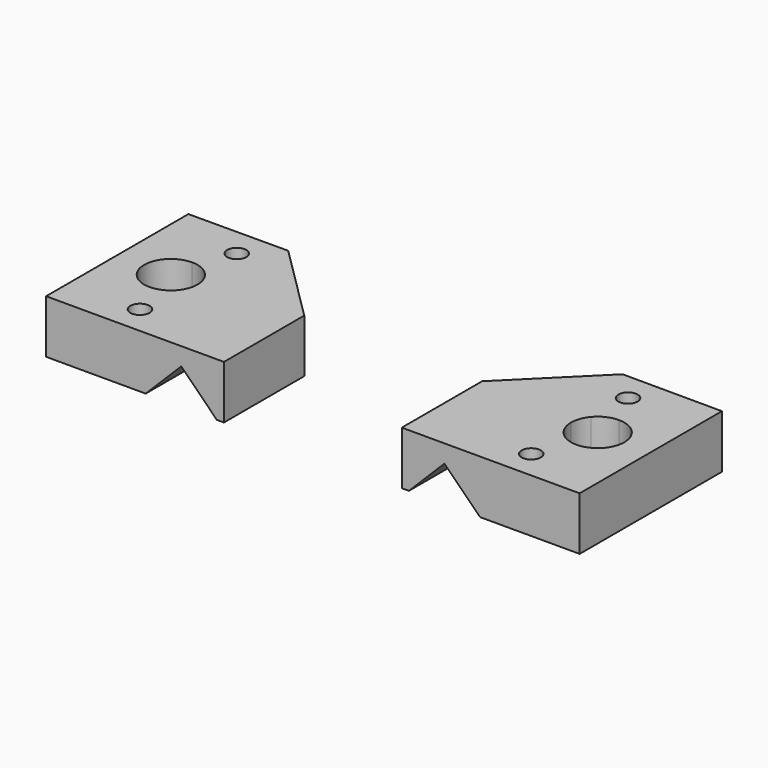
from build123d import *

# Parameters (mm, degrees)
F1_DEPTH  = 15
F3_DEPTH  = 50.1607448159
F4_R      = 4
F5_DEPTH  = 10
F7_DEPTH  = 15.001
F9_D      = 5.4
F9_DEPTH  = 60
F9_TIP    = 1.6223236714
F11_DEPTH = 15.001


with BuildPart() as f1:
    # F0 (on Top) → F1 (new body)
    with BuildSketch(Plane.XY):
        Polygon((24.6076433315, -30.0955416439), (24.6076433315, 20.064203172), (-25.3923566685, 19.9044583561), (-25.3923566685, -30.0955416439), align=None)
    extrude(amount=F1_DEPTH)

    # F2 (on face) → F3 (cut, through all)
    with BuildSketch(Plane.XZ.offset(30.0955416439)):
        Polygon((2.6076433315, 0), (22.6076433315, 0), (12.6076433315, 10), align=None)
    extrude(amount=-F3_DEPTH, mode=Mode.SUBTRACT)

    # F4 (on face) → F5 (cut)
    with BuildSketch(Plane(origin=(0, 0, 0), x_dir=(1, 0, 0), z_dir=(0, 0, -1))):
        with Locations((-17.3923566685, 22.0955416439)):
            Circle(F4_R)
        with Locations((-17.3923566685, -11.9044583561)):
            Circle(F4_R)
    extrude(amount=-F5_DEPTH, mode=Mode.SUBTRACT)

    # F6 (on face) → F7 (cut, through all)
    with BuildSketch(Plane(origin=(0, 0, 0), x_dir=(1, 0, 0), z_dir=(0, 0, -1))):
        with BuildLine():
            Line((-10.3923566685, 5), (-10.3923566685, 12.5))
            ThreePointArc((-10.3923566685, 12.5), (-17.8923566685, 5), (-10.3923566685, -2.5))
            Line((-10.3923566685, -2.5), (-10.3923566685, 5))
        make_face()
        with BuildLine():
            ThreePointArc((-2.8923566685, 5), (-5.0890558096, 10.3033008589), (-10.3923566685, 12.5))
            Line((-10.3923566685, 12.5), (-10.3923566685, 5))
            Line((-10.3923566685, 5), (-4.6306970715, 0.1986170025))
            ThreePointArc((-4.6306970715, 0.1986170025), (-3.3403198359, 2.4468105219), (-2.8923566685, 5))
        make_face()
        with BuildLine():
            Line((-4.6306970715, 0.1986170025), (-10.3923566685, 5))
            Line((-10.3923566685, 5), (-10.3923566685, -2.5))
            ThreePointArc((-10.3923566685, -2.5), (-7.2111911966, -1.7919206592), (-4.6306970715, 0.1986170025))
        make_face()
    extrude(amount=-F7_DEPTH, mode=Mode.SUBTRACT)

    # F9
    with Locations(Plane.XY.offset(15)):
        with Locations((-5.3923566685, -22.0955416439), (-5.3923566685, 11.9044583561)):
            Hole(F9_D / 2, depth=F9_DEPTH)
            with Locations((0, 0, -(F9_DEPTH + F9_TIP / 2))):  # 118° drill point
                Cone(0, F9_D / 2, F9_TIP, mode=Mode.SUBTRACT)

    # F10 (on face) → F11 (cut, through all)
    with BuildSketch(Plane(origin=(0, 0, 0), x_dir=(1, 0, 0), z_dir=(0, 0, -1))):
        Polygon((27.6873877408, 4.9260849556), (2.6076433315, -19.993915453), (27.6075157405, -20.0737874533), align=None)
    extrude(amount=-F11_DEPTH, mode=Mode.SUBTRACT)


with BuildPart() as f12_1:
    # F12: instance of F1
    add(f1.part.mirror(Plane(origin=(24.6076433315, -15.9807492232, 7.5), x_dir=(0, 1, 0), z_dir=(1, 0, 0))))


with BuildPart() as f12_1_1:
    # F13: moved
    add(f12_1.part.moved(Location((50, 0, 0))))


solid = Compound([f1.part, f12_1_1.part])
